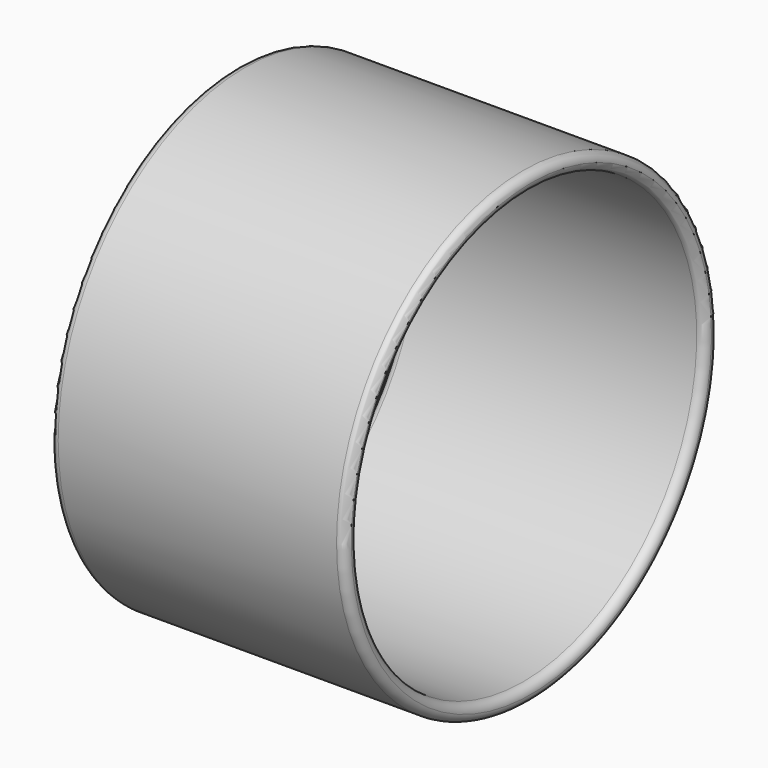
from build123d import *

# Parameters (mm, degrees)
F0_W = 18
F0_H = 1
F2_R = 0.49999
F3_R = 0.49999


# Not quite as in the source:
# - a fillet or chamfer is up to 0.001 mm smaller than in the source, because OpenCascade refuses the exact size


with BuildPart() as f1:
    # F0 (on Front) → F1 (revolve)
    with BuildSketch(Plane.XZ):
        with Locations((-9, 13.75)):
            Rectangle(F0_W, F0_H)
    revolve(axis=Axis((-8.2086159056, 0, 0), (1, 0, 0)))

    # F2 (radius 0.5 in the source; OpenCascade refuses exactly that, so slightly less here)
    f2_edges = [f1.edges().sort_by_distance(p)[0] for p in [
        (0, 0, -13.25),
        (0, 0, -14.25),
    ]]
    fillet(f2_edges, radius=F2_R)

    # F3 (radius 0.5 in the source; OpenCascade refuses exactly that, so slightly less here)
    f3_edges = [f1.edges().sort_by_distance(p)[0] for p in [
        (-18, 0, -14.25),
        (-18, 0, -13.25),
    ]]
    fillet(f3_edges, radius=F3_R)


solid = f1.part
